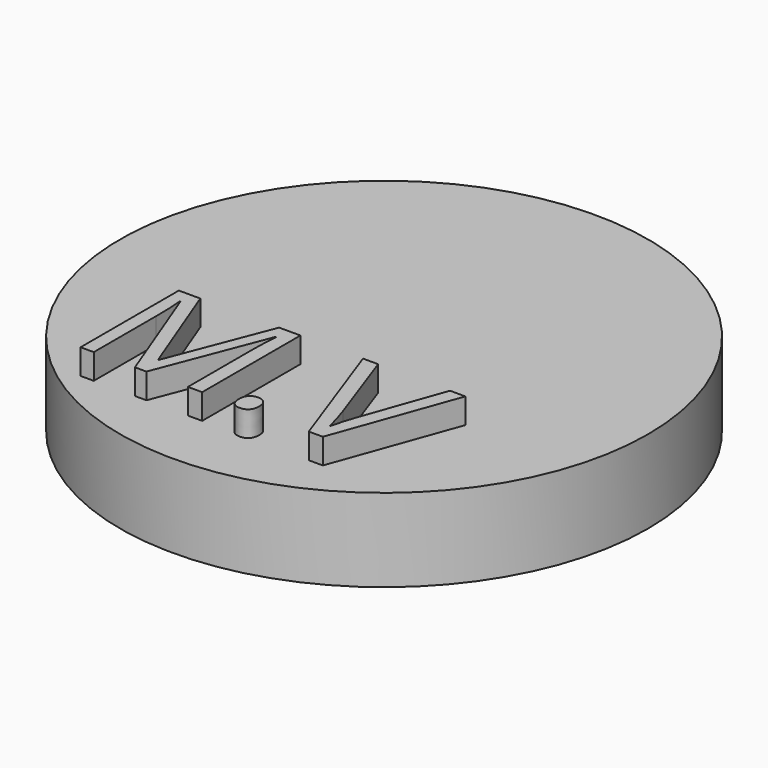
from build123d import *

# Parameters (mm, degrees)
F1_R         = 18.568241068
F3_DEPTH     = 5.842
F8_TEXT_SIZE = 12.0995715002
F9_DEPTH     = 7.62


# Not quite as in the source:
# - a feature of the source that left no trace in its solid (it failed there, or was rolled back) is left out
# - the program builds the solid bodies; features that only make, move or delete a surface that nothing else refers to are left out
# - Text() gives the source's letters only with a copy of the font that has no kerning and outlines rounded to 1/6400 em; it was checked with that copy


with BuildPart() as f3:
    # F1 (on face) → F3 (new body)
    with BuildSketch(Plane.XY):
        Circle(F1_R)
    extrude(amount=F3_DEPTH)

    # F8 (on Top) → F9 (join)
    with BuildSketch(Plane.XY):
        with Locations((-11.2957758829, -14.0531095676)):
            Text('M.V', F8_TEXT_SIZE, font='Open Sans', text_align=(TextAlign.LEFT, TextAlign.BOTTOM))
    extrude(amount=F9_DEPTH)


solid = f3.part
